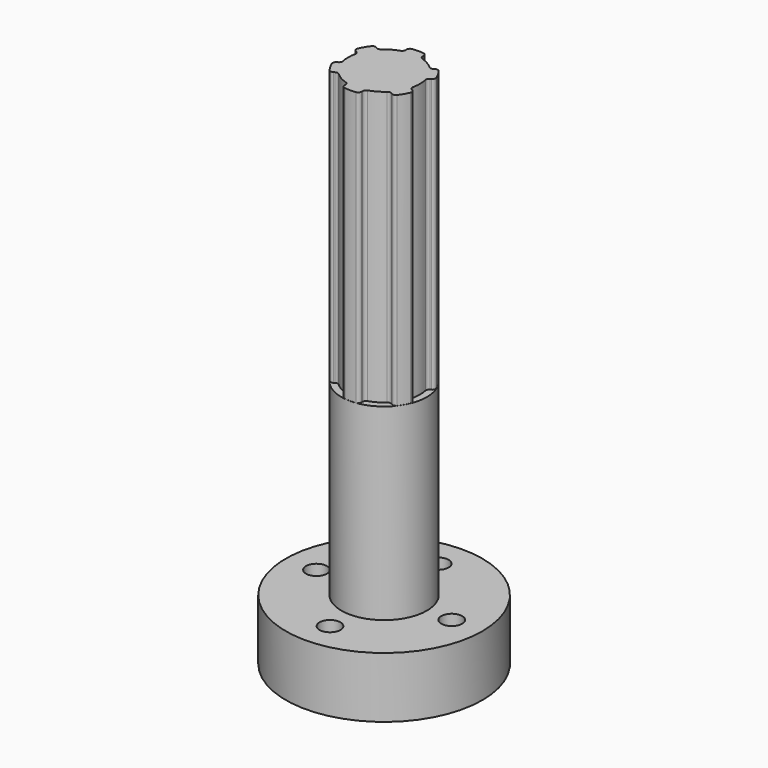
from build123d import *

# Parameters (mm, degrees)
F0_R             = 14.605
F1_DEPTH         = 9.017
F2_R             = 6.35
F3_DEPTH         = 27.94
F4_R             = 5.334
F5_DEPTH         = 40.64
F6_R             = 8.255
F7_DEPTH         = 2.3
F8_R             = 5.06
F9_DEPTH         = 4.1
F11_D            = 3.1
F13_DEPTH        = 40.64
F13_COPIES_COUNT = 6
F14_R            = 0.508


# Not quite as in the source:
# - a pattern or mirror of a feature is missing from the dataset's text; its kind, count and spacing are read off the source's solid


with BuildPart() as f1:
    # F0 (on Top) → F1 (new body)
    with BuildSketch(Plane.XY):
        Circle(F0_R)
    extrude(amount=F1_DEPTH)

    # F2 (on face) → F3 (join)
    with BuildSketch(Plane.XY.offset(9.017)):
        Circle(F2_R)
    extrude(amount=F3_DEPTH)

    # F4 (on face) → F5 (join)
    with BuildSketch(Plane.XY.offset(36.957)):
        Circle(F4_R)
    extrude(amount=F5_DEPTH)

    # F6 (on face) → F7 (cut)
    with BuildSketch(Plane(origin=(0, 0, 0), x_dir=(1, 0, 0), z_dir=(0, 0, -1))):
        Circle(F6_R)
    extrude(amount=-F7_DEPTH, mode=Mode.SUBTRACT)

    # F8 (on face) → F9 (cut)
    with BuildSketch(Plane(origin=(0, 0, 0), x_dir=(1, 0, 0), z_dir=(0, 0, -1))):
        Circle(F8_R)
    extrude(amount=-F9_DEPTH, mode=Mode.SUBTRACT)

    # F11 (through all)
    with Locations(Plane.XY.offset(9.017)):
        with Locations((0, -10.05), (-10.05, 0), (0, 10.05), (10.05, 0)):
            Hole(F11_D / 2)

    # F12 (on face) → F13 (join, through all)
    with BuildSketch(Plane.XY.offset(77.597)):
        with BuildLine():
            Line((-1.27, -5.1806038258), (-1.27, -6.1957780109))
            ThreePointArc((-1.27, -6.1957780109), (0, -6.3246), (1.27, -6.1957780109))
            Line((1.27, -6.1957780109), (1.27, -5.1806038258))
            ThreePointArc((1.27, -5.1806038258), (0, -5.334), (-1.27, -5.1806038258))
        make_face()
    f13 = extrude(amount=-F13_DEPTH)

    # F13_copies: F13 ×6 about axis
    f13_copies_axis = Axis((0, 0, 0), (0, 0, 1))
    for i in range(1, F13_COPIES_COUNT):
        add(f13.rotate(f13_copies_axis, i * 360 / F13_COPIES_COUNT))

    # F14
    f14_edges = [f1.edges().sort_by_distance(p)[0] for p in [
        (1.27, -6.195778, 57.277),
        (1.27, -5.180604, 57.277),
        (-1.27, -6.195778, 57.277),
        (-1.27, -5.180604, 57.277),
        (3.851535, -3.690154, 57.277),
        (4.730701, -4.197741, 57.277),
        (6.000701, -1.998037, 57.277),
        (5.121535, -1.49045, 57.277),
        (5.121535, 1.49045, 57.277),
        (6.000701, 1.998037, 57.277),
        (4.730701, 4.197741, 57.277),
        (3.851535, 3.690154, 57.277),
        (1.27, 5.180604, 57.277),
        (1.27, 6.195778, 57.277),
        (-1.27, 6.195778, 57.277),
        (-1.27, 5.180604, 57.277),
        (-3.851535, 3.690154, 57.277),
        (-4.730701, 4.197741, 57.277),
        (-6.000701, 1.998037, 57.277),
        (-5.121535, 1.49045, 57.277),
        (-5.121535, -1.49045, 57.277),
        (-6.000701, -1.998037, 57.277),
        (-4.730701, -4.197741, 57.277),
        (-3.851535, -3.690154, 57.277),
    ]]
    fillet(f14_edges, radius=F14_R)


solid = f1.part
